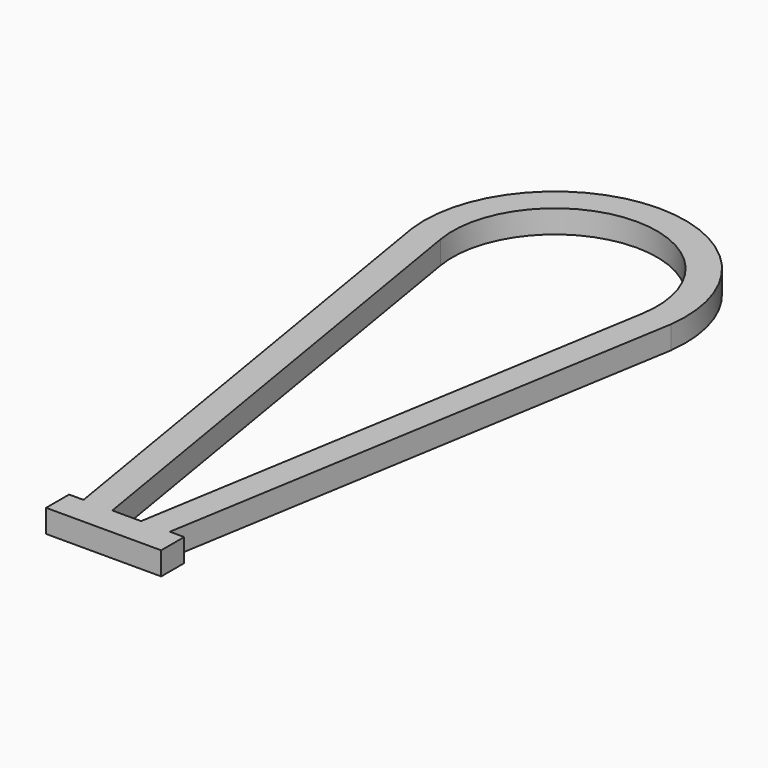
from build123d import *

# Parameters (mm, degrees)
F1_DEPTH = 4


# Not quite as in the source:
# - ends of sketch curves that miss each other by under 0.0002 mm in the source are joined


with BuildPart() as f1:
    # F0 (on Top) → F1 (new body)
    with BuildSketch(Plane.XY):
        with BuildLine():
            Line((-2.4992633137, 15), (-17.5086315699, 105.0827546296))
            ThreePointArc((-17.5086315699, 105.0827546296), (0, 125.75), (17.5086315699, 105.0827546296))
            Line((17.5086315699, 105.0827546296), (2.4992633137, 15))
            Line((2.4992633137, 15), (7.4992633137, 14.9999997765))
            Line((7.4992633137, 14.9999997765), (22.5086315699, 105.0827546296))
            ThreePointArc((22.5086315699, 105.0827546296), (0, 130.6968900006), (-22.5086315699, 105.0827546296))
            Line((-22.5086315699, 105.0827546296), (-7.4992633137, 15))
            Line((-7.4992633137, 15), (-2.4992633137, 15))
        make_face()
        Polygon((2.4992633137, 14.9999997765), (-2.4992633137, 14.9999997765), (-7.4992633137, 14.9999997765), (-10.0086377934, 14.9999997765), (-10.0086377934, 9.9999997765), (9.9913622066, 9.9999997765), (9.9913622066, 14.9999997765), (7.4992633137, 14.9999997765), align=None)
    extrude(amount=F1_DEPTH)


solid = f1.part
